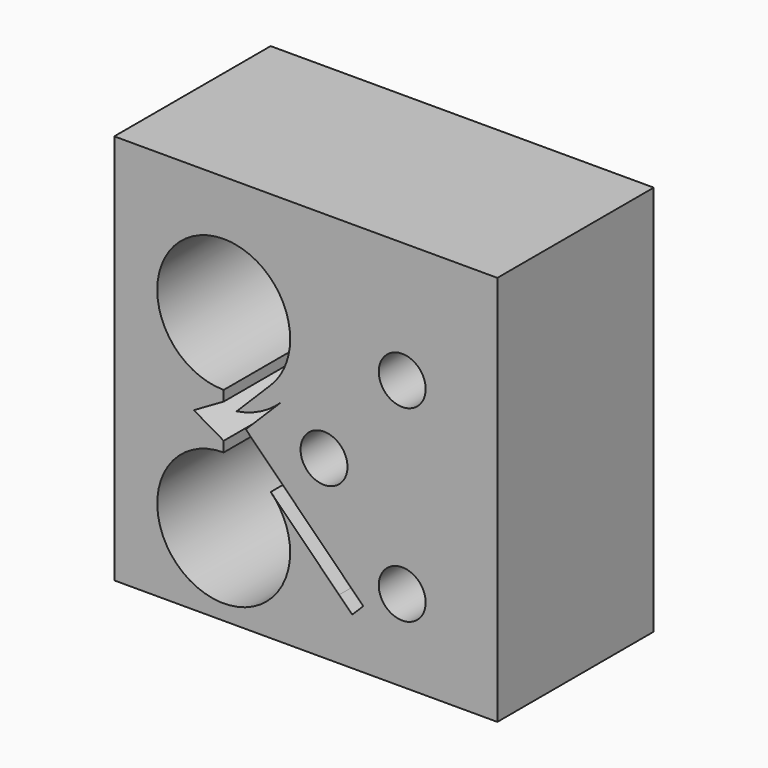
from build123d import *

# Parameters (mm, degrees)
F1_DEPTH = 25
F0_R     = 3
F2_DEPTH = 25


# Not quite as in the source:
# - ends of sketch curves that miss each other by under 0.0002 mm in the source are joined


with BuildPart() as f1:
    # F0 (on Front) → F1 (new body)
    with BuildSketch(Plane.XZ):
        with BuildLine():
            ThreePointArc((-35.5724336391, 25.151316084), (-36.2194536929, 21.8985163721), (-38.0620115133, 19.1409229296))
            Line((-38.0620115133, 19.1409229296), (-40.551597873, 16.6513245695))
            Line((-40.551597873, 16.6513245695), (-42.4208999514, 14.7820134806))
            ThreePointArc((-42.4208999514, 14.7820134806), (-39.3014754977, 15.797816289), (-36.6477945425, 17.7267127756))
            ThreePointArc((-36.6477945425, 17.7267127756), (-34.0584132659, 28.3087511137), (-42.2491526952, 35.491801885))
            ThreePointArc((-42.2491526952, 35.491801885), (-43.1573109451, 35.6113615168), (-44.0724336391, 35.651316084))
            Line((-44.0724336391, 35.651316084), (-44.0724336391, 33.651316084))
            ThreePointArc((-44.0724336391, 33.651316084), (-43.3316200297, 33.6189719105), (-42.5964443036, 33.5221855419))
            ThreePointArc((-42.5964443036, 33.5221855419), (-37.5610624566, 30.6150186129), (-35.5724336391, 25.151316084))
        make_face()
    extrude(amount=F1_DEPTH)

    # F0 (on Front) → F2 (join)
    with BuildSketch(Plane.XZ):
        with BuildLine():
            Line((-44.0724072079, 15.3363250258), (-44.0724107491, 16.651316084))
            ThreePointArc((-44.0724107491, 16.651316084), (-52.5724336391, 25.151304639), (-44.0724336391, 33.651316084))
            Line((-44.0724336391, 33.651316084), (-44.0724336391, 35.651316084))
            Line((-44.0724336391, 35.651316084), (-44.0724336391, 40.651316084))
            Line((-44.0724336391, 40.651316084), (-58.0724336391, 40.651316084))
            Line((-58.0724336391, 40.651316084), (-58.0722360097, 19.007240245))
            Line((-58.0722360097, 19.007240245), (-47.893068168, 13.1304188771))
            Line((-47.893068168, 13.1304188771), (-44.0724072079, 15.3363250258))
        make_face()
        Polygon((-18.7646776515, 35.6099158673), (-36.6477945425, 17.7267127756), (-41.2439775428, 13.1305076206), (-26.2214527658, -1.8919447448), (-18.7646776515, -9.348683916), (-9.0724336391, -9.348683916), (-9.0724336391, 35.6099158673), align=None)
        with Locations((-21.2439775428, 1.1096808038)):
            Circle(F0_R, mode=Mode.SUBTRACT)
        with Locations((-31.2439775428, 13.1305076206)):
            Circle(F0_R, mode=Mode.SUBTRACT)
        with Locations((-21.2439775428, 25.1513302219)):
            Circle(F0_R, mode=Mode.SUBTRACT)
        with BuildLine():
            ThreePointArc((-42.2491526952, 35.491801885), (-34.0584132659, 28.3087511137), (-36.6477945425, 17.7267127756))
            Line((-36.6477945425, 17.7267127756), (-18.7646776515, 35.6099158673))
            Line((-18.7646776515, 35.6099158673), (-9.0724336391, 35.6099158673))
            Line((-9.0724336391, 35.6099158673), (-9.0724336391, 40.651316084))
            Line((-9.0724336391, 40.651316084), (-18.7646776515, 40.651316084))
            Line((-18.7646776515, 40.651316084), (-44.0724336391, 40.651316084))
            Line((-44.0724336391, 40.651316084), (-44.0724336391, 35.651316084))
            ThreePointArc((-44.0724336391, 35.651316084), (-43.1573109451, 35.6113615168), (-42.2491526952, 35.491801885))
        make_face()
        with BuildLine():
            Line((-44.0723953274, 10.9245988987), (-47.893068168, 13.1304188771))
            Line((-47.893068168, 13.1304188771), (-58.0721286869, 7.2534116208))
            Line((-58.0721286869, 7.2534116208), (-58.0719770953, -9.348683916))
            Line((-58.0719770953, -9.348683916), (-21.593111593, -9.348683916))
            Line((-21.593111593, -9.348683916), (-27.6356629198, -3.3061617156))
            Line((-27.6356629198, -3.3061617156), (-29.3171299504, -1.62470279))
            Line((-29.3171299504, -1.62470279), (-38.061976782, 7.1201018897))
            ThreePointArc((-38.061976782, 7.1201018897), (-36.2193967899, 4.3624994422), (-35.5723688964, 1.1096808038))
            ThreePointArc((-35.5723688964, 1.1096808038), (-50.0827684437, -4.9007349291), (-44.0723917864, 9.6096808038))
            Line((-44.0723917864, 9.6096808038), (-44.0723953274, 10.9245988987))
        make_face()
        Polygon((-58.0721286869, 7.2534116208), (-47.893068168, 13.1304188771), (-58.0722360097, 19.007240245), align=None)
        Polygon((-18.7646776515, -9.348683916), (-26.2214527658, -1.8919447448), (-27.6356629198, -3.3061617156), (-21.593111593, -9.348683916), align=None)
    extrude(amount=F2_DEPTH)


solid = f1.part
